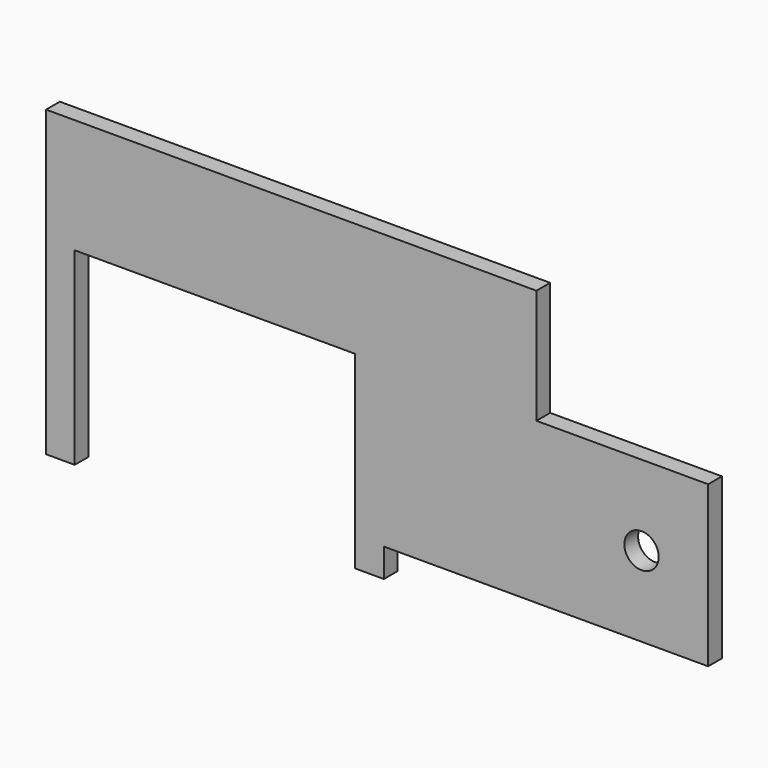
from build123d import *

# Parameters (mm, degrees)
F0_W     = 49
F0_H     = 20
F0_W_2   = 5
F0_H_2   = 33
F0_H_3   = 28
F0_H_4   = 5
F0_W_3   = 26.6433528662
F0_W_4   = 30
F0_R     = 3
F1_DEPTH = 3


# Not quite as in the source:
# - a feature names something its author has since deleted; it is built from what else it names


with BuildPart() as f1:
    # F0 (on Front) → F1 (new body)
    with BuildSketch(Plane.XZ):
        with Locations((29.5, 10)):
            Rectangle(F0_W, F0_H)
        with Locations((2.5, 10)):
            Rectangle(F0_W_2, F0_H)
        with Locations((2.5, -16.5)):
            Rectangle(F0_W_2, F0_H_2)
        with Locations((56.5, 10)):
            Rectangle(F0_W_2, F0_H)
        with Locations((56.5, -14)):
            Rectangle(F0_W_2, F0_H_3)
        with Locations((56.5, -30.5)):
            Rectangle(F0_W_2, F0_H_4)
        with Locations((72.3216764331, -14)):
            Rectangle(F0_W_3, F0_H_3)
        with Locations((72.3216764331, 10)):
            Rectangle(F0_W_3, F0_H)
        with Locations((100.6433528662, -14)):
            Rectangle(F0_W_4, F0_H_3)
        with Locations((104, -14)):
            Circle(F0_R, mode=Mode.SUBTRACT)
    extrude(amount=F1_DEPTH)


solid = f1.part
